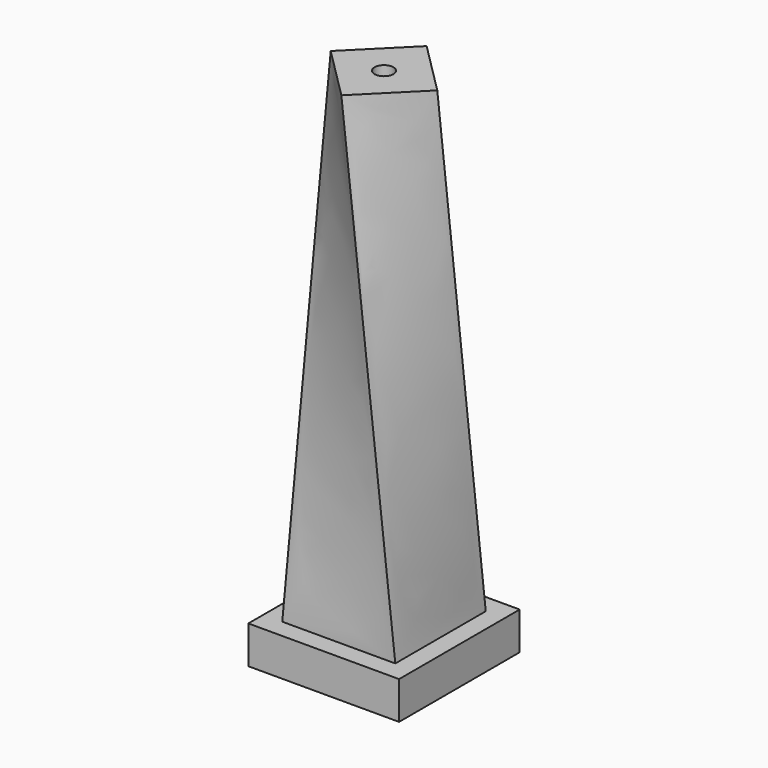
from build123d import *

# Parameters (mm, degrees)
F0_W     = 101.6
F0_H     = 101.6
F0_W_2   = 76.2
F0_H_2   = 76.2
F1_DEPTH = 25.4
F2_W     = 76.2
F2_H     = 76.2
F6_D     = 19.05
F6_DEPTH = 76.2
F6_TIP   = 5.7231973962
F7_D     = 12.7
F7_DEPTH = 38.1
F7_TIP   = 3.8154649308


with BuildPart() as f1:
    # F0 (on Top) → F1 (new body)
    with BuildSketch(Plane.XY):
        with Locations((-1.3143327087, 25.9222988339)):
            Rectangle(F0_W, F0_H)
        with Locations((-1.3143327087, 25.9222988339)):
            Rectangle(F0_W_2, F0_H_2, mode=Mode.SUBTRACT)
        with Locations((-1.3143327087, 25.9222988339)):
            Rectangle(F0_W_2, F0_H_2)
    extrude(amount=F1_DEPTH)

    # F2 (on face) → F5 section 0
    with BuildSketch(Plane.XY.offset(25.4)):
        with Locations((-1.3143327087, 25.9222988339)):
            Rectangle(F2_W, F2_H)
    # F4 (on offset) → F5 section 1
    with BuildSketch(Plane.XY.offset(349.25)):
        Polygon((-1.3143327087, -9.9987256503), (34.6066917756, 25.9222988339), (-1.3143327087, 61.8433233182), (-37.235357193, 25.9222988339), align=None)
    loft()

    # F6
    with Locations(Plane(origin=(0, 0, 0), x_dir=(1, 0, 0), z_dir=(0, 0, -1))):
        with Locations((-1.3143327087, -25.9222988339)):
            Hole(F6_D / 2, depth=F6_DEPTH)
            with Locations((0, 0, -(F6_DEPTH + F6_TIP / 2))):  # 118° drill point
                Cone(0, F6_D / 2, F6_TIP, mode=Mode.SUBTRACT)

    # F7
    with Locations(Plane.XY.offset(349.25)):
        with Locations((-1.3143327087, 25.9222988339)):
            Hole(F7_D / 2, depth=F7_DEPTH)
            with Locations((0, 0, -(F7_DEPTH + F7_TIP / 2))):  # 118° drill point
                Cone(0, F7_D / 2, F7_TIP, mode=Mode.SUBTRACT)


solid = f1.part
